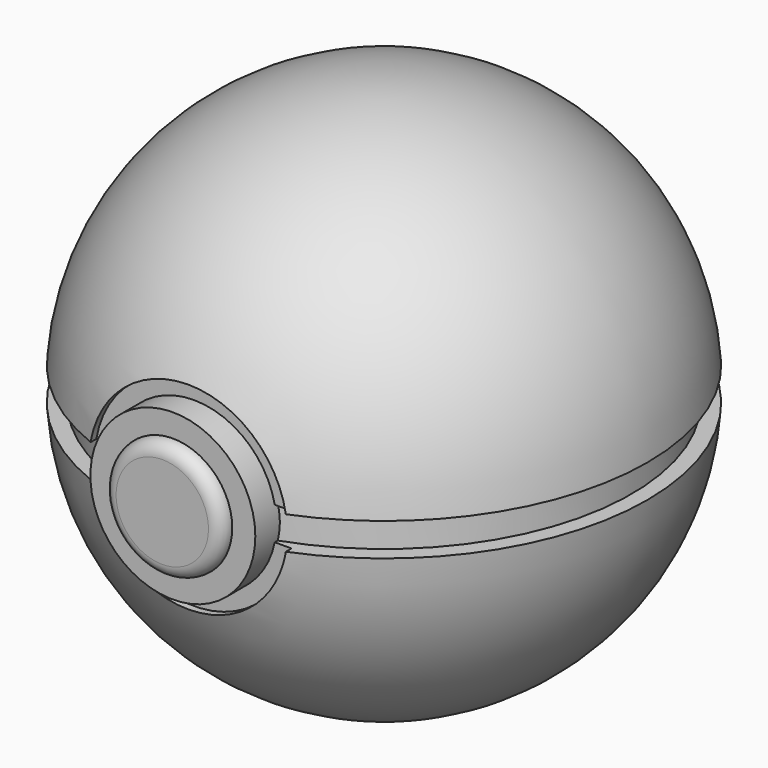
from build123d import *

# Parameters (mm, degrees)
F2_R     = 12.5
F3_DEPTH = 40
F4_R     = 15
F4_R_2   = 12.5
F5_DEPTH = 4
F6_R     = 9
F7_DEPTH = 2
F8_R     = 1.99999


# Not quite as in the source:
# - a fillet or chamfer is up to 0.001 mm smaller than in the source, because OpenCascade refuses the exact size


with BuildPart() as f1:
    # F0 (on Front) → F1 (revolve)
    with BuildSketch(Plane.XZ):
        with BuildLine():
            Line((0, 40), (0, -40))
            ThreePointArc((0, -40), (27.3861278753, -29.1547594742), (39.9217985567, -2.5))
            Line((39.9217985567, -2.5), (37.5, -2.5))
            Line((37.5, -2.5), (37.5, 0))
            Line((37.5, 0), (37.5, 2.5))
            Line((37.5, 2.5), (39.9217985567, 2.5))
            ThreePointArc((39.9217985567, 2.5), (27.3861278753, 29.1547594742), (0, 40))
        make_face()
    revolve(axis=Axis((0, 0, 0), (0, 0, -1)))

    # F2 (on Front) → F3 (join)
    with BuildSketch(Plane.XZ):
        Circle(F2_R)
    extrude(amount=F3_DEPTH)

    # F4 (on face) → F5 (cut)
    with BuildSketch(Plane.XZ.offset(40)):
        Circle(F4_R)
        Circle(F4_R_2, mode=Mode.SUBTRACT)
    extrude(amount=-F5_DEPTH, mode=Mode.SUBTRACT)

    # F6 (on face) → F7 (join)
    with BuildSketch(Plane.XZ.offset(40)):
        Circle(F6_R)
    extrude(amount=F7_DEPTH)

    # F8 (radius 2 in the source; OpenCascade refuses exactly that, so slightly less here)
    f8_edges = [f1.edges().sort_by_distance(p)[0] for p in [
        (-9, -42, 0),
    ]]
    fillet(f8_edges, radius=F8_R)


solid = f1.part
